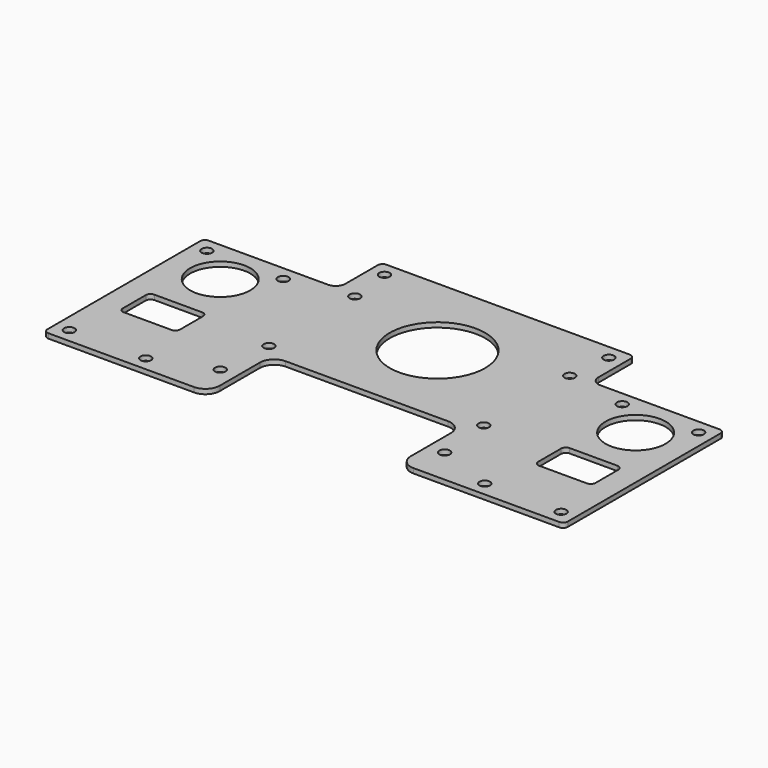
from build123d import *

# Parameters (mm, degrees)
F0_W     = 109
F0_H     = 70
F0_R     = 1.1
F0_R_2   = 6.3
F1_DEPTH = 1
F2_W     = 53
F2_H     = 10.5
F3_DEPTH = 1
F5_DEPTH = 1
F6_R     = 1
F7_R     = 1.1
F7_W     = 40
F7_H     = 16.5
F7_R_2   = 10
F8_DEPTH = 1
F9_R     = 3


# Not quite as in the source:
# - a feature names something its author has since deleted; it is built from what else it names


with BuildPart() as f1:
    # F0 (on Top) → F1 (new body)
    with BuildSketch(Plane.XY):
        Rectangle(F0_W, F0_H)
        with Locations((-51.5, -26)):
            Circle(F0_R, mode=Mode.SUBTRACT)
        with Locations((-35.5, -26)):
            Circle(F0_R, mode=Mode.SUBTRACT)
        with Locations((-23.5, -21.5)):
            Circle(F0_R, mode=Mode.SUBTRACT)
        with BuildLine():
            ThreePointArc((-37.5, -14.5), (-37.7928932188, -15.2071067812), (-38.5, -15.5))
            Line((-38.5, -15.5), (-48.5, -15.5))
            ThreePointArc((-48.5, -15.5), (-49.2071067812, -15.2071067812), (-49.5, -14.5))
            Line((-49.5, -14.5), (-49.5, -8.5))
            ThreePointArc((-49.5, -8.5), (-49.2071067812, -7.7928932188), (-48.5, -7.5))
            Line((-48.5, -7.5), (-38.5, -7.5))
            ThreePointArc((-38.5, -7.5), (-37.7928932188, -7.7928932188), (-37.5, -8.5))
            Line((-37.5, -8.5), (-37.5, -14.5))
        make_face(mode=Mode.SUBTRACT)
        with Locations((23.5, -21.5)):
            Circle(F0_R, mode=Mode.SUBTRACT)
        with Locations((35.5, -26)):
            Circle(F0_R, mode=Mode.SUBTRACT)
        with Locations((51.5, -26)):
            Circle(F0_R, mode=Mode.SUBTRACT)
        with BuildLine():
            Line((38.5, -7.5), (48.5, -7.5))
            ThreePointArc((48.5, -7.5), (49.2071067812, -7.7928932188), (49.5, -8.5))
            Line((49.5, -8.5), (49.5, -14.5))
            ThreePointArc((49.5, -14.5), (49.2071067812, -15.2071067812), (48.5, -15.5))
            Line((48.5, -15.5), (38.5, -15.5))
            ThreePointArc((38.5, -15.5), (37.7928932188, -15.2071067812), (37.5, -14.5))
            Line((37.5, -14.5), (37.5, -8.5))
            ThreePointArc((37.5, -8.5), (37.7928932188, -7.7928932188), (38.5, -7.5))
        make_face(mode=Mode.SUBTRACT)
        with Locations((-43.5, 3.5)):
            Circle(F0_R_2, mode=Mode.SUBTRACT)
        with Locations((-51.5, 10)):
            Circle(F0_R, mode=Mode.SUBTRACT)
        with Locations((-35.5, 10)):
            Circle(F0_R, mode=Mode.SUBTRACT)
        with Locations((-23.5, 21.5)):
            Circle(F0_R, mode=Mode.SUBTRACT)
        with Locations((43.5, 3.5)):
            Circle(F0_R_2, mode=Mode.SUBTRACT)
        with Locations((35.5, 10)):
            Circle(F0_R, mode=Mode.SUBTRACT)
        with Locations((51.5, 10)):
            Circle(F0_R, mode=Mode.SUBTRACT)
        with Locations((23.5, 21.5)):
            Circle(F0_R, mode=Mode.SUBTRACT)
    extrude(amount=F1_DEPTH)

    # F2 (on face) → F3 (cut, through all)
    with BuildSketch(Plane.XY.offset(1)):
        with BuildLine():
            Line((-26.5, 35), (-54.5, 35))
            Line((-54.5, 35), (-54.5, 13))
            Line((-54.5, 13), (-28.5, 13))
            ThreePointArc((-28.5, 13), (-27.0857864376, 13.5857864376), (-26.5, 15))
            Line((-26.5, 15), (-26.5, 24.5))
            Line((-26.5, 24.5), (-26.5, 35))
        make_face()
        with Locations((0, 29.75)):
            Rectangle(F2_W, F2_H)
        with BuildLine():
            Line((54.5, 35), (26.5, 35))
            Line((26.5, 35), (26.5, 24.5))
            Line((26.5, 24.5), (26.5, 15))
            ThreePointArc((26.5, 15), (27.0857864376, 13.5857864376), (28.5, 13))
            Line((28.5, 13), (54.5, 13))
            Line((54.5, 13), (54.5, 35))
        make_face()
    extrude(amount=-F3_DEPTH, mode=Mode.SUBTRACT)

    # F4 (on face) → F5 (cut, through all)
    with BuildSketch(Plane.XY.offset(1)):
        Polygon((-54.5, -29), (-54.5, -35), (0, -35), (54.5, -35), (54.5, -29), (0, -29), align=None)
    extrude(amount=-F5_DEPTH, mode=Mode.SUBTRACT)

    # F6
    f6_edges = [f1.edges().sort_by_distance(p)[0] for p in [
        (-54.5, -29, 0.5),
        (54.5, -29, 0.5),
        (54.5, 13, 0.5),
        (26.5, 24.5, 0.5),
        (-26.5, 24.5, 0.5),
        (-54.5, 13, 0.5),
    ]]
    fillet(f6_edges, radius=F6_R)

    # F7 (on face) → F8 (cut, through all)
    with BuildSketch(Plane.XY.offset(1)):
        with Locations((-22.5, -10)):
            Circle(F7_R)
        with Locations((22.5, -10)):
            Circle(F7_R)
        with Locations((-22.5, 12.5)):
            Circle(F7_R)
        with Locations((22.5, 12.5)):
            Circle(F7_R)
        with Locations((0, -20.75)):
            Rectangle(F7_W, F7_H)
        with Locations((0, 6)):
            Circle(F7_R_2)
    extrude(amount=-F8_DEPTH, mode=Mode.SUBTRACT)

    # F9
    f9_edges = [f1.edges().sort_by_distance(p)[0] for p in [
        (-20, -29, 0.5),
        (-20, -12.5, 0.5),
        (20, -12.5, 0.5),
        (20, -29, 0.5),
    ]]
    fillet(f9_edges, radius=F9_R)


solid = f1.part
